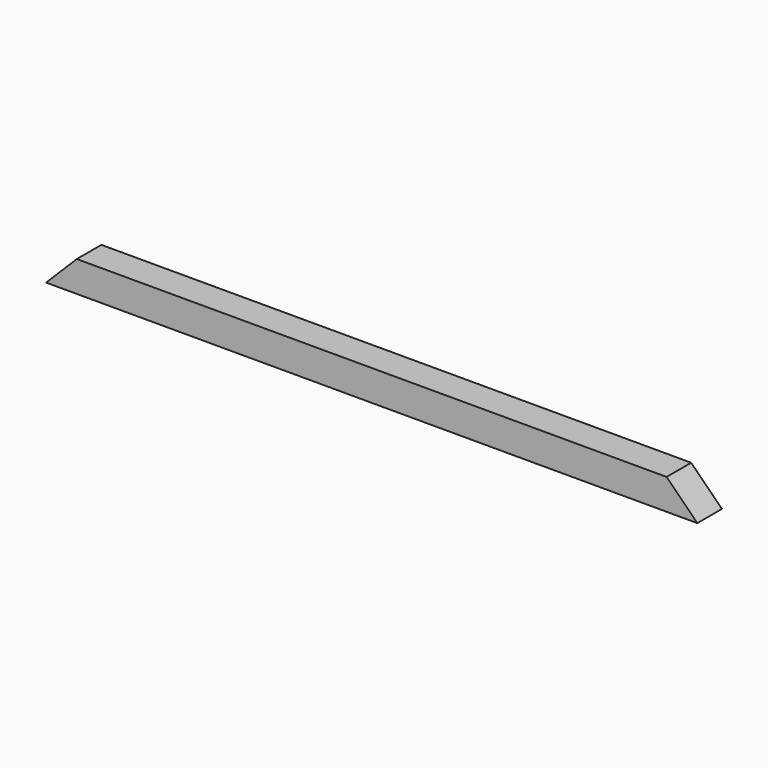
from build123d import *

# Parameters (mm, degrees)
F0_W     = 211.9884
F0_H     = 9.99998
F1_DEPTH = 9.99998
F2_SIZE  = 9.99997
F3_SIZE  = 9.99997


# Not quite as in the source:
# - a fillet or chamfer is up to 0.001 mm smaller than in the source, because OpenCascade refuses the exact size


with BuildPart() as f1:
    # F0 (on Front) → F1 (new body)
    with BuildSketch(Plane.XZ):
        with Locations((35.5700679509, -8.0864099948)):
            Rectangle(F0_W, F0_H)
    extrude(amount=F1_DEPTH)

    # F2 (size 9.99998 in the source; OpenCascade refuses exactly that, so slightly less here)
    f2_edges = [f1.edges().sort_by_distance(p)[0] for p in [
        (141.564268, -4.99999, -3.08642),
    ]]
    chamfer(f2_edges, length=F2_SIZE)

    # F3 (size 9.99998 in the source; OpenCascade refuses exactly that, so slightly less here)
    f3_edges = [f1.edges().sort_by_distance(p)[0] for p in [
        (-70.424132, -4.99999, -3.08642),
    ]]
    chamfer(f3_edges, length=F3_SIZE)


solid = f1.part
